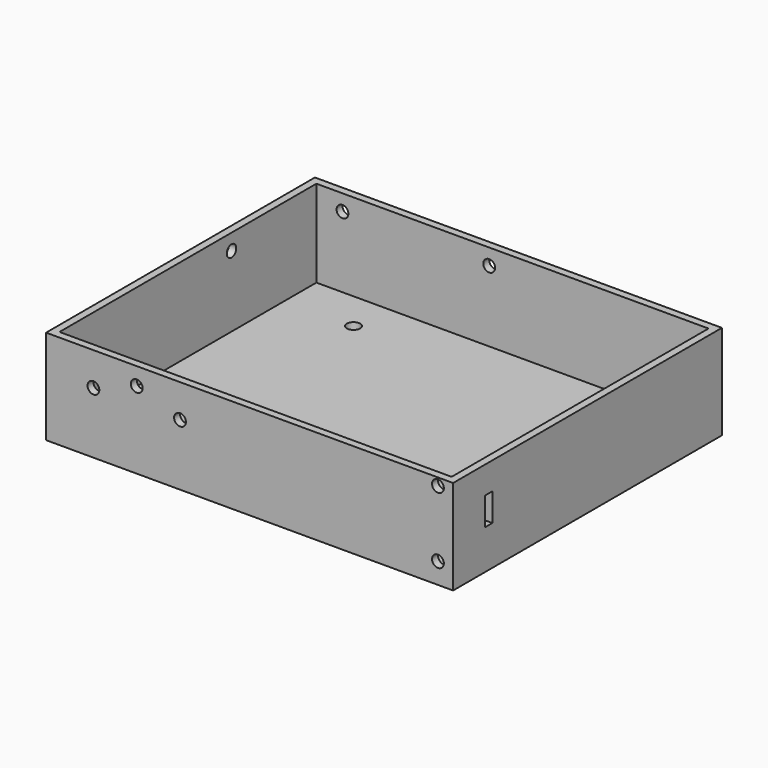
from build123d import *

# Parameters (mm, degrees)
F0_W      = 109.22
F0_H      = 25.4
F1_DEPTH  = 90.17
F2_W      = 105.22204
F2_H      = 86.17204
F3_DEPTH  = 23.368
F6_D      = 3.556
F10_R     = 2.7904831324
F11_DEPTH = 25.4
F13_D     = 3.175
F13_DEPTH = 12.7
F13_TIP   = 0.9538662327
F14_W     = 2.5
F14_H     = 7.5
F15_DEPTH = 5.08
F17_D     = 3.175
F17_DEPTH = 12.7
F17_TIP   = 0.9538662327
F19_D     = 3.175
F19_DEPTH = 12.7
F19_TIP   = 0.9538662327
F21_D     = 3.175
F21_DEPTH = 12.7
F21_TIP   = 0.9538662327


# Not quite as in the source:
# - a feature of the source that left no trace in its solid (it failed there, or was rolled back) is left out
# - a feature names something its author has since deleted; it is built from what else it names


with BuildPart() as f1:
    # F0 (on Front) → F1 (new body)
    with BuildSketch(Plane.XZ):
        Rectangle(F0_W, F0_H)
    extrude(amount=F1_DEPTH)

    # F2 (on face) → F3 (cut)
    with BuildSketch(Plane.XY.offset(12.7)):
        with Locations((0, -45.085)):
            Rectangle(F2_W, F2_H)
    extrude(amount=-F3_DEPTH, mode=Mode.SUBTRACT)

    # F6 (through all)
    with Locations(Plane.XY.offset(-10.668)):
        with Locations((-34.2227290702, -12.5292580739), (31.5179094365, -9.3542580739), (31.5179094365, -57.6142580739)):
            Hole(F6_D / 2)

    # F10 (on face) → F11 (cut)
    with BuildSketch(Plane(origin=(0, 0, -12.7), x_dir=(1, 0, 0), z_dir=(0, 0, -1))):
        with Locations((-37.1684581041, 13.9195527881)):
            Circle(F10_R)
    extrude(amount=F11_DEPTH, mode=Mode.SUBTRACT)

    # F13
    with Locations(Plane.XZ.offset(90.17)):
        with Locations((50.546, 10.668), (50.546, -7.112)):
            Hole(F13_D / 2, depth=F13_DEPTH)
            with Locations((0, 0, -(F13_DEPTH + F13_TIP / 2))):  # 118° drill point
                Cone(0, F13_D / 2, F13_TIP, mode=Mode.SUBTRACT)

    # F14 (on face) → F15 (cut)
    with BuildSketch(Plane.YZ.offset(54.61)):
        with Locations((-78.2630409374, 1.6418104)):
            Rectangle(F14_W, F14_H)
    extrude(amount=-F15_DEPTH, mode=Mode.SUBTRACT)

    # F17
    with Locations(Plane(origin=(0, 0, 0), x_dir=(1, 0, 0), z_dir=(0, 1, 0))):
        with Locations((-6.2431572373, -8.382), (-45.6131572373, -8.382)):
            Hole(F17_D / 2, depth=F17_DEPTH)
            with Locations((0, 0, -(F17_DEPTH + F17_TIP / 2))):  # 118° drill point
                Cone(0, F17_D / 2, F17_TIP, mode=Mode.SUBTRACT)

    # F19
    with Locations(Plane(origin=(-54.61, 0, 0), x_dir=(0, -1, 0), z_dir=(-1, 0, 0))):
        with Locations((30.48, 8.382)):
            Hole(F19_D / 2, depth=F19_DEPTH)
            with Locations((0, 0, -(F19_DEPTH + F19_TIP / 2))):  # 118° drill point
                Cone(0, F19_D / 2, F19_TIP, mode=Mode.SUBTRACT)

    # F21
    with Locations(Plane.XZ.offset(90.17)):
        with Locations((-30.2895, 8.001), (-41.91, 3.7953188), (-18.669, 3.7953188)):
            Hole(F21_D / 2, depth=F21_DEPTH)
            with Locations((0, 0, -(F21_DEPTH + F21_TIP / 2))):  # 118° drill point
                Cone(0, F21_D / 2, F21_TIP, mode=Mode.SUBTRACT)


solid = f1.part
